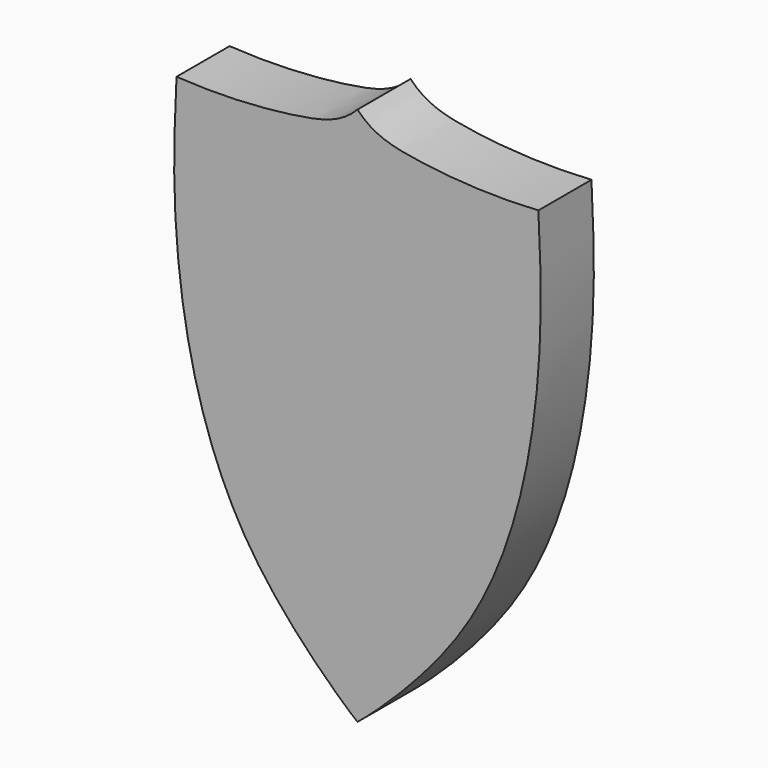
from build123d import *

# Parameters (mm, degrees)
F3_DEPTH = 25.4


with BuildPart() as f3:
    # F2 (on Front) → F3 (new body)
    with BuildSketch(Plane.XZ):
        with BuildLine():
            add(Edge.make_bspline(
                [(852.3174320221, -579.0984034538), (858.2559670769, -585.2658680133), (874.7004180149, -589.5600168599), (903.3677973809, -591.7229662034), (921.5745517731, -590.548992157)],
                knots=[0, 0, 0, 0, 0.4124822499, 1, 1, 1, 1], degree=3))
            add(Edge.make_bspline(
                [(852.3174320221, -579.0984034538), (846.3788969673, -585.2658680133), (829.9344460293, -589.5600168599), (801.2670666633, -591.7229662034), (783.0603122711, -590.548992157)],
                knots=[0, 0, 0, 0, 0.4124822499, 1, 1, 1, 1], degree=3))
            add(Edge.make_bspline(
                [(783.0603122711, -590.548992157), (782.310067677, -607.0117239943), (780.3337231664, -645.9329231025), (797.0494904139, -738.7160589782), (849.2076784238, -783.028401487), (852.3174320221, -785.4467630386)],
                knots=[0, 0, 0, 0, 0.2826716235, 0.666214736, 0.9677866144, 0.9677866144, 0.9677866144, 0.9677866144], degree=3))
            add(Edge.make_bspline(
                [(921.5745517731, -590.548992157), (922.3247963672, -607.0117239943), (924.3011408777, -645.9329231025), (907.5853736303, -738.7160589782), (855.4271856204, -783.028401487), (852.3174320221, -785.4467630386)],
                knots=[0, 0, 0, 0, 0.2826716235, 0.666214736, 0.9677866144, 0.9677866144, 0.9677866144, 0.9677866144], degree=3))
        make_face()
    extrude(amount=F3_DEPTH)


solid = f3.part
